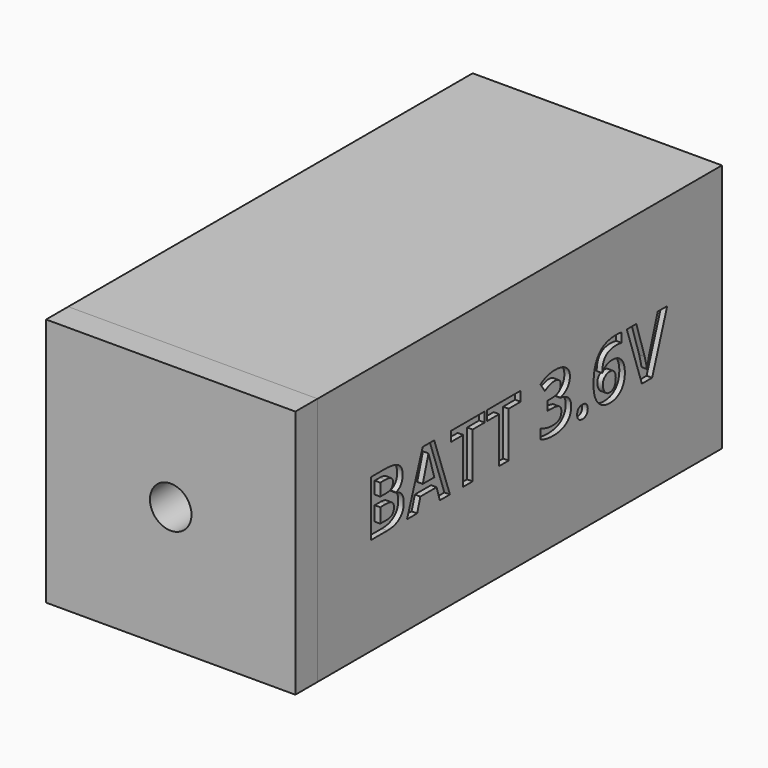
from build123d import *

# Parameters (mm, degrees)
F0_W          = 18
F0_H          = 18
F1_DEPTH      = 36.5
F2_T          = -1.5
F3_W          = 14.4989397377
F3_H          = 14.4989397377
F4_DEPTH      = 1
F6_W          = 18
F6_H          = 18
F7_DEPTH      = 2
F8_R          = 1.5
F9_DEPTH      = 3
F10_TEXT_SIZE = 5.6120096512
F11_DEPTH     = 0.4


# Not quite as in the source:
# - Text() gives the source's letters only with a copy of the font that has no kerning and outlines rounded to 1/6400 em; it was checked with that copy


with BuildPart() as f1:
    # F0 (on Front) → F1 (new body)
    with BuildSketch(Plane.XZ):
        Rectangle(F0_W, F0_H)
    extrude(amount=F1_DEPTH)

    # F2
    f2_openings = [f1.faces().sort_by_distance(p)[0] for p in [
        (0, -36.5, 0),
    ]]
    offset(amount=F2_T, openings=f2_openings)

    # F10 (on face) → F11 (cut)
    with BuildSketch(Plane.YZ.offset(9)):
        with Locations((-32.1923345327, -1.9431809196)):
            Text('BATT 3.6V', F10_TEXT_SIZE, font='Open Sans', font_style=FontStyle.BOLD, text_align=(TextAlign.LEFT, TextAlign.BOTTOM))
    extrude(amount=-F11_DEPTH, mode=Mode.SUBTRACT)


with BuildPart() as f4:
    # F3 (on face) → F4 (new body)
    with BuildSketch(Plane.XZ.offset(36.5)):
        Rectangle(F3_W, F3_H)
    extrude(amount=-F4_DEPTH)

    # F6 (on face) → F7 (join)
    with BuildSketch(Plane.XZ.offset(36.5)):
        Rectangle(F6_W, F6_H)
    extrude(amount=F7_DEPTH)

    # F8 (on face) → F9 (cut, through all)
    with BuildSketch(Plane.XZ.offset(38.5)):
        Circle(F8_R)
    extrude(amount=-F9_DEPTH, mode=Mode.SUBTRACT)


solid = Compound([f1.part, f4.part])
